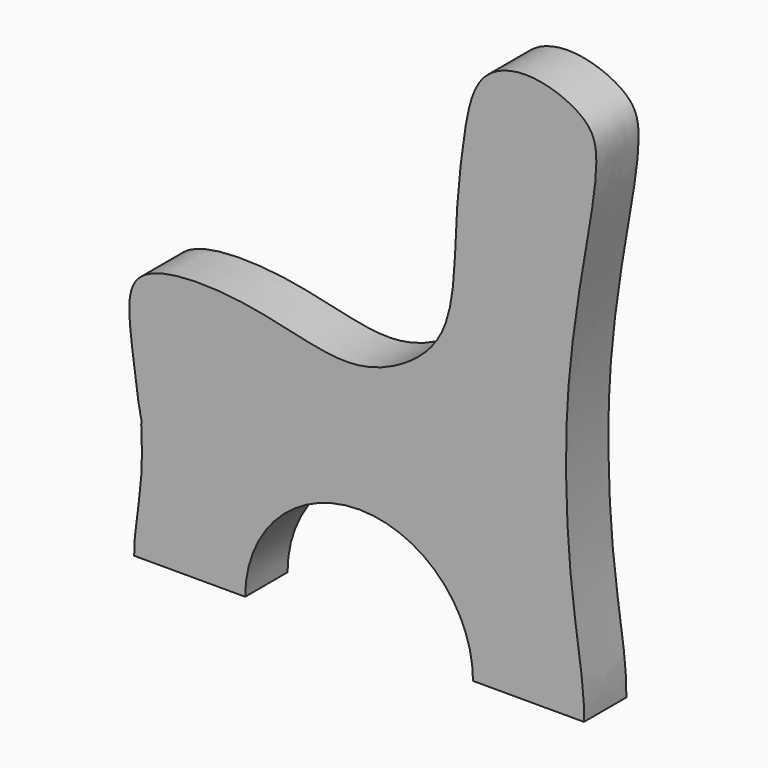
from build123d import *

# Parameters (mm, degrees)
F1_DEPTH = 100


# Not quite as in the source:
# - a feature names something its author has since deleted; it is built from what else it names


with BuildPart() as f1:
    # F0 (on Front) → F1 (new body)
    with BuildSketch(Plane.XZ):
        with BuildLine():
            add(Edge.make_bspline(
                [(-107.1904016608, 223.0619813646), (-105.9979918183, 196.1607068759), (-103.4859317579, 139.4875607748), (-120.6546638515, 33.1554072128), (-120.4633990058, 8.6219013235), (-120.3961820889, 0)],
                knots=[0, 0, 0, 0, 0.3694955634, 0.7784194782, 1, 1, 1, 1], degree=3))
            Line((-120.3961820889, 0), (89.193292446, 0))
            ThreePointArc((89.193292446, 0), (304.3673823213, 215.1740898753), (519.5414721966, 0))
            Line((519.5414721966, 0), (729.1309467315, 0))
            add(Edge.make_bspline(
                [(729.1309467315, 0), (730.6280350069, 33.114385577), (718.9435659416, 122.3793674346), (699.9952566475, 244.8674798388), (688.2222079991, 505.9964295412), (725.3780292604, 754.7645456461), (761.4925243229, 943.711566112), (737.5601770429, 1009.1502839125), (627.5496486471, 1053.2939418875), (524.0869903868, 1020.947495576), (500.1715872211, 896.4642389354), (484.6756036033, 745.5335457472), (484.638859196, 556.5561535268), (377.5624440027, 470.4861770143), (264.8516251268, 439.5025609935), (94.5921509343, 498.8003261332), (-136.5586315251, 496.9574954182), (-128.9627521746, 370.8298243446), (-114.2454774135, 271.691381961), (-110.7910852201, 245.6909311455), (-104.7735227724, 223.501382532), (-107.1904016608, 223.0619813646)],
                knots=[0, 0, 0, 0, 0.0472990962, 0.0968195061, 0.1670734157, 0.2391114884, 0.2982144094, 0.3319616778, 0.3775848729, 0.4199988556, 0.4665643231, 0.5221378989, 0.581086589, 0.6296272862, 0.6750654507, 0.735360656, 0.7965294542, 0.8399260459, 0.883894523, 0.9079125847, 0.9266071202, 0.9266071202, 0.9266071202, 0.9266071202], degree=3))
        make_face()
    extrude(amount=F1_DEPTH)


solid = f1.part
